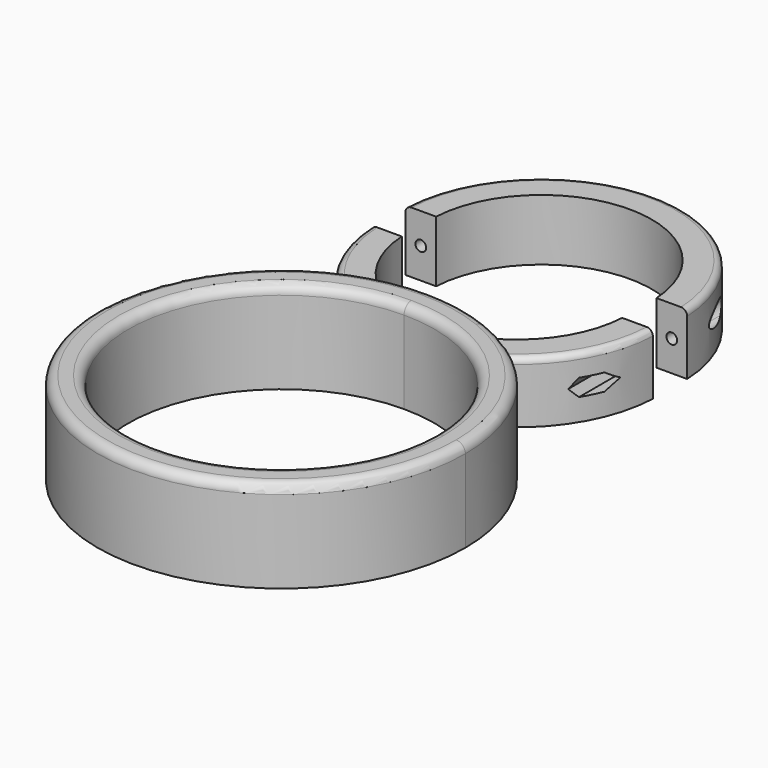
from build123d import *

# Parameters (mm, degrees)
F1_DEPTH       = 20
F2_DEPTH       = 30
F3_R           = 1.75
F4_DEPTH       = 23.9
F5_DEPTH       = 25
F6_DEPTH       = 4
F7_R           = 1.75
F8_DEPTH       = 25
F9_DEPTH       = 25
F10_DEPTH      = 7
F11_R          = 3
F12_T4_ANGLE   = 71.0644406489
F12_S5_R       = 60
F12_T6_DEPTH   = 31
F12_T10_ANGLE  = 71.0644406489
F12_S11_R      = 60
F12_T12_DEPTH  = 31
F12_2_T2_ANGLE = 187.4907274343


# Not quite as in the source:
# - a fillet or chamfer that OpenCascade refuses, or shapes differently, is made with other operations: its cross-section is extruded or revolved along the edge and cut away or added


with BuildPart() as f1:
    # F0 (on Top) → F1 (new body)
    with BuildSketch(Plane.XY):
        with BuildLine():
            ThreePointArc((-2.47e-08, 60), (11.3192314105, 58.9226187493), (22.2319585876, 55.7291666667))
            ThreePointArc((22.2319585876, 55.7291666667), (39.0970674362, 71.763265115), (45.9565011723, 94))
            Line((45.9565011723, 94), (35.9444015112, 94))
            ThreePointArc((35.9444015112, 94), (24.7386337447, 69.8466063303), (-2.47e-08, 60))
        make_face()
    extrude(amount=F1_DEPTH)



with BuildPart() as f1b:
    # F0 (on Top) → F1, piece 2 (new body)
    with BuildSketch(Plane.XY):
        with BuildLine():
            ThreePointArc((-45.9565011723, 94), (-39.0970674362, 71.763265115), (-22.2319585876, 55.7291666667))
            ThreePointArc((-22.2319585876, 55.7291666667), (-11.3192314348, 58.9226187446), (-2.47e-08, 60))
            ThreePointArc((-2.47e-08, 60), (-24.7386337627, 69.8466063473), (-35.9444015112, 94))
            Line((-35.9444015112, 94), (-45.9565011723, 94))
        make_face()
    extrude(amount=F1_DEPTH)


with BuildPart() as f1c:
    # F0 (on Top) → F1, piece 3 (new body)
    with BuildSketch(Plane.XY):
        with BuildLine():
            Line((35.9444015112, 108), (45.9565011723, 108))
            ThreePointArc((45.9565011723, 108), (0, 152), (-45.9565011723, 108))
            Line((-45.9565011723, 108), (-35.9444015112, 108))
            ThreePointArc((-35.9444015112, 108), (0, 142), (35.9444015112, 108))
        make_face()
    extrude(amount=F1_DEPTH)

    # F7 (on face) → F8 (cut)
    with BuildSketch(Plane.XZ.offset(-108)):
        with Locations((-40.9504513418, 10)):
            Circle(F7_R)
        with Locations((40.9504513418, 10)):
            Circle(F7_R)
    extrude(amount=-F8_DEPTH, mode=Mode.SUBTRACT)

    # F7 (on face) → F9 (cut)
    with BuildSketch(Plane.XZ.offset(-108)):
        with BuildLine():
            Line((-39.4004513418, 12.6846787517), (-37.8504513418, 10))
            ThreePointArc((-37.8504513418, 10), (-38.26577259, 11.55), (-39.4004513418, 12.6846787517))
        make_face()
        Polygon((-42.5004513418, 7.3153212483), (-39.4004513418, 7.3153212483), (-37.8504513418, 10), (-39.4004513418, 12.6846787517), (-42.5004513418, 12.6846787517), (-44.0504513418, 10), align=None)
        with Locations((-40.9504513418, 10)):
            Circle(F7_R, mode=Mode.SUBTRACT)
        with BuildLine():
            Line((-42.5004513418, 12.6846787517), (-39.4004513418, 12.6846787517))
            ThreePointArc((-39.4004513418, 12.6846787517), (-40.9504513418, 13.1), (-42.5004513418, 12.6846787517))
        make_face()
        with BuildLine():
            ThreePointArc((-42.5004513418, 12.6846787517), (-43.6351300935, 11.55), (-44.0504513418, 10))
            Line((-44.0504513418, 10), (-42.5004513418, 12.6846787517))
        make_face()
        with BuildLine():
            ThreePointArc((-44.0504513418, 10), (-43.6351300935, 8.45), (-42.5004513418, 7.3153212483))
            Line((-42.5004513418, 7.3153212483), (-44.0504513418, 10))
        make_face()
        with BuildLine():
            ThreePointArc((-42.5004513418, 7.3153212483), (-40.9504513418, 6.9), (-39.4004513418, 7.3153212483))
            Line((-39.4004513418, 7.3153212483), (-42.5004513418, 7.3153212483))
        make_face()
        with BuildLine():
            Line((-37.8504513418, 10), (-39.4004513418, 7.3153212483))
            ThreePointArc((-39.4004513418, 7.3153212483), (-38.26577259, 8.45), (-37.8504513418, 10))
        make_face()
        with BuildLine():
            Line((37.8504513418, 10), (39.4004513418, 12.6846787517))
            ThreePointArc((39.4004513418, 12.6846787517), (38.26577259, 11.55), (37.8504513418, 10))
        make_face()
        Polygon((44.0504513418, 10), (42.5004513418, 12.6846787517), (39.4004513418, 12.6846787517), (37.8504513418, 10), (39.4004513418, 7.3153212483), (42.5004513418, 7.3153212483), align=None)
        with Locations((40.9504513418, 10)):
            Circle(F7_R, mode=Mode.SUBTRACT)
        with BuildLine():
            Line((39.4004513418, 12.6846787517), (42.5004513418, 12.6846787517))
            ThreePointArc((42.5004513418, 12.6846787517), (40.9504513418, 13.1), (39.4004513418, 12.6846787517))
        make_face()
        with BuildLine():
            ThreePointArc((44.0504513418, 10), (43.6351300935, 11.55), (42.5004513418, 12.6846787517))
            Line((42.5004513418, 12.6846787517), (44.0504513418, 10))
        make_face()
        with BuildLine():
            ThreePointArc((42.5004513418, 7.3153212483), (43.6351300935, 8.45), (44.0504513418, 10))
            Line((44.0504513418, 10), (42.5004513418, 7.3153212483))
        make_face()
        with BuildLine():
            Line((39.4004513418, 7.3153212483), (37.8504513418, 10))
            ThreePointArc((37.8504513418, 10), (38.26577259, 8.45), (39.4004513418, 7.3153212483))
        make_face()
        with BuildLine():
            ThreePointArc((39.4004513418, 7.3153212483), (40.9504513418, 6.9), (42.5004513418, 7.3153212483))
            Line((42.5004513418, 7.3153212483), (39.4004513418, 7.3153212483))
        make_face()
    extrude(amount=-F9_DEPTH, mode=Mode.SUBTRACT)

    # F7 (on face) → F10 (join)
    with BuildSketch(Plane.XZ.offset(-108)):
        Polygon((44.0504513418, 10), (42.5004513418, 12.6846787517), (39.4004513418, 12.6846787517), (37.8504513418, 10), (39.4004513418, 7.3153212483), (42.5004513418, 7.3153212483), align=None)
        with Locations((40.9504513418, 10)):
            Circle(F7_R, mode=Mode.SUBTRACT)
        with BuildLine():
            Line((37.8504513418, 10), (39.4004513418, 12.6846787517))
            ThreePointArc((39.4004513418, 12.6846787517), (38.26577259, 11.55), (37.8504513418, 10))
        make_face()
        with BuildLine():
            Line((39.4004513418, 7.3153212483), (37.8504513418, 10))
            ThreePointArc((37.8504513418, 10), (38.26577259, 8.45), (39.4004513418, 7.3153212483))
        make_face()
        with BuildLine():
            ThreePointArc((39.4004513418, 7.3153212483), (40.9504513418, 6.9), (42.5004513418, 7.3153212483))
            Line((42.5004513418, 7.3153212483), (39.4004513418, 7.3153212483))
        make_face()
        with BuildLine():
            ThreePointArc((42.5004513418, 7.3153212483), (43.6351300935, 8.45), (44.0504513418, 10))
            Line((44.0504513418, 10), (42.5004513418, 7.3153212483))
        make_face()
        with BuildLine():
            ThreePointArc((44.0504513418, 10), (43.6351300935, 11.55), (42.5004513418, 12.6846787517))
            Line((42.5004513418, 12.6846787517), (44.0504513418, 10))
        make_face()
        with BuildLine():
            Line((39.4004513418, 12.6846787517), (42.5004513418, 12.6846787517))
            ThreePointArc((42.5004513418, 12.6846787517), (40.9504513418, 13.1), (39.4004513418, 12.6846787517))
        make_face()
        with BuildLine():
            Line((-39.4004513418, 12.6846787517), (-37.8504513418, 10))
            ThreePointArc((-37.8504513418, 10), (-38.26577259, 11.55), (-39.4004513418, 12.6846787517))
        make_face()
        Polygon((-42.5004513418, 7.3153212483), (-39.4004513418, 7.3153212483), (-37.8504513418, 10), (-39.4004513418, 12.6846787517), (-42.5004513418, 12.6846787517), (-44.0504513418, 10), align=None)
        with Locations((-40.9504513418, 10)):
            Circle(F7_R, mode=Mode.SUBTRACT)
        with BuildLine():
            Line((-37.8504513418, 10), (-39.4004513418, 7.3153212483))
            ThreePointArc((-39.4004513418, 7.3153212483), (-38.26577259, 8.45), (-37.8504513418, 10))
        make_face()
        with BuildLine():
            ThreePointArc((-42.5004513418, 7.3153212483), (-40.9504513418, 6.9), (-39.4004513418, 7.3153212483))
            Line((-39.4004513418, 7.3153212483), (-42.5004513418, 7.3153212483))
        make_face()
        with BuildLine():
            ThreePointArc((-44.0504513418, 10), (-43.6351300935, 8.45), (-42.5004513418, 7.3153212483))
            Line((-42.5004513418, 7.3153212483), (-44.0504513418, 10))
        make_face()
        with BuildLine():
            ThreePointArc((-42.5004513418, 12.6846787517), (-43.6351300935, 11.55), (-44.0504513418, 10))
            Line((-44.0504513418, 10), (-42.5004513418, 12.6846787517))
        make_face()
        with BuildLine():
            Line((-42.5004513418, 12.6846787517), (-39.4004513418, 12.6846787517))
            ThreePointArc((-39.4004513418, 12.6846787517), (-40.9504513418, 13.1), (-42.5004513418, 12.6846787517))
        make_face()
    extrude(amount=-F10_DEPTH)

    # F12#2: fillet of radius 2 on 1 edges, made by hand

    # F12_2_s1 → F12_2_t2 (revolve, cut)
    with BuildSketch(Plane(origin=(6.909384127, 105.5476965336, 0), x_dir=(0, 0, 1), z_dir=(-0.0653223839, -0.9978642123, 0))):
        with BuildLine():
            ThreePointArc((18, -39.07582731), (19.4142135624, -38.4900408724), (20, -37.07582731))
            Line((20, -37.07582731), (20, -39.07582731))
            Line((20, -39.07582731), (18, -39.07582731))
        make_face()
    revolve(axis=Axis((0, 106, 20), (0, 0, 1)), revolution_arc=F12_2_T2_ANGLE, mode=Mode.SUBTRACT)


with BuildPart() as f1_1:
    add(f1.part)

    add(f1b.part)  # F2 merges F1b
    # F0 (on Top) → F2 (join)
    with BuildSketch(Plane.XY):
        with BuildLine():
            ThreePointArc((22.2319585876, 55.7291666667), (11.4791477819, 51.4553127051), (4.18e-08, 50))
            ThreePointArc((4.18e-08, 50), (-11.4791477414, 51.4553126946), (-22.2319585876, 55.7291666667))
            ThreePointArc((-22.2319585876, 55.7291666667), (-33.6606779845, -49.668488578), (60, 0))
            ThreePointArc((60, 0), (49.668488578, 33.6606779845), (22.2319585876, 55.7291666667))
        make_face()
        with BuildLine():
            ThreePointArc((4.18e-08, 50), (35.3553390741, 35.3553390445), (50, 0))
            ThreePointArc((50, 0), (-35.3553390741, -35.3553390445), (4.18e-08, 50))
        make_face(mode=Mode.SUBTRACT)
        with BuildLine():
            ThreePointArc((-22.2319585876, 55.7291666667), (-11.4791477414, 51.4553126946), (4.18e-08, 50))
            ThreePointArc((4.18e-08, 50), (11.4791477819, 51.4553127051), (22.2319585876, 55.7291666667))
            ThreePointArc((22.2319585876, 55.7291666667), (11.3192314105, 58.9226187493), (-2.47e-08, 60))
            ThreePointArc((-2.47e-08, 60), (-11.3192314348, 58.9226187446), (-22.2319585876, 55.7291666667))
        make_face()
    extrude(amount=F2_DEPTH)

    # F3 (on face) → F4 (cut)
    with BuildSketch(Plane(origin=(0, 94, 0), x_dir=(-1, 0, 0), z_dir=(0, 1, 0))):
        with Locations((-40.9504513418, 10)):
            Circle(F3_R)
        with Locations((40.9504513418, 10)):
            Circle(F3_R)
    extrude(amount=-F4_DEPTH, mode=Mode.SUBTRACT)

    # F3 (on face) → F5 (cut)
    with BuildSketch(Plane(origin=(0, 94, 0), x_dir=(-1, 0, 0), z_dir=(0, 1, 0))):
        Polygon((-42.5504513418, 7.2287187079), (-39.3504513418, 7.2287187079), (-37.7504513418, 10), (-39.3504513418, 12.7712812921), (-42.5504513418, 12.7712812921), (-44.1504513418, 10), align=None)
        with Locations((-40.9504513418, 10)):
            Circle(F3_R, mode=Mode.SUBTRACT)
        Polygon((42.5504513418, 12.7712812921), (39.3504513418, 12.7712812921), (37.7504513418, 10), (39.3504513418, 7.2287187079), (42.5504513418, 7.2287187079), (44.1504513418, 10), align=None)
        with Locations((40.9504513418, 10)):
            Circle(F3_R, mode=Mode.SUBTRACT)
    extrude(amount=-F5_DEPTH, mode=Mode.SUBTRACT)

    # F3 (on face) → F6 (join)
    with BuildSketch(Plane(origin=(0, 94, 0), x_dir=(-1, 0, 0), z_dir=(0, 1, 0))):
        Polygon((-42.5504513418, 7.2287187079), (-39.3504513418, 7.2287187079), (-37.7504513418, 10), (-39.3504513418, 12.7712812921), (-42.5504513418, 12.7712812921), (-44.1504513418, 10), align=None)
        with Locations((-40.9504513418, 10)):
            Circle(F3_R, mode=Mode.SUBTRACT)
        Polygon((42.5504513418, 12.7712812921), (39.3504513418, 12.7712812921), (37.7504513418, 10), (39.3504513418, 7.2287187079), (42.5504513418, 7.2287187079), (44.1504513418, 10), align=None)
        with Locations((40.9504513418, 10)):
            Circle(F3_R, mode=Mode.SUBTRACT)
    extrude(amount=-F6_DEPTH)

    # F11
    f11_edges = [f1_1.edges().sort_by_distance(p)[0] for p in [
        (-22.231959, -55.729167, 30),
        (0, -50, 30),
    ]]
    fillet(f11_edges, radius=F11_R)

    # F12: fillet of radius 2 on 2 edges, made by hand


with BuildPart() as f12_tool2:
    # F12_s3 → F12_t4 (revolve)
    with BuildSketch(Plane(origin=(34.1449001636, 14.2638799975, 0), x_dir=(0, 0, 1), z_dir=(-0.9227230986, -0.3854634656, 0))):
        with BuildLine():
            ThreePointArc((18, 42.5814174657), (19.4142135624, 43.1672039033), (20, 44.5814174657))
            Line((20, 44.5814174657), (20, 42.5814174657))
            Line((20, 42.5814174657), (18, 42.5814174657))
        make_face()
    revolve(axis=Axis((0, 96, 20), (0, 0, 1)), revolution_arc=F12_T4_ANGLE)

    # F12_s5 → F12_t6 (cut, symmetric)
    with BuildSketch(Plane.XY.offset(19)):
        Circle(F12_S5_R)
    extrude(amount=F12_T6_DEPTH, both=True, mode=Mode.SUBTRACT)


with BuildPart() as f1_2:
    add(f1_1.part)

    # F12_t1: cut F12_tool2
    add(f12_tool2.part, mode=Mode.SUBTRACT)


with BuildPart() as f12_tool8:
    # F12_s9 → F12_t10 (revolve)
    with BuildSketch(Plane(origin=(6.243588842, 95.5922010247, 0), x_dir=(0, 0, 1), z_dir=(0.0651759618, 0.9978737866, 0))):
        with BuildLine():
            ThreePointArc((18, -52.2568923302), (19.4142135624, -51.6711058926), (20, -50.2568923302))
            Line((20, -50.2568923302), (20, -52.2568923302))
            Line((20, -52.2568923302), (18, -52.2568923302))
        make_face()
    revolve(axis=Axis((0, 96, 20), (0, 0, 1)), revolution_arc=F12_T10_ANGLE)

    # F12_s11 → F12_t12 (cut, symmetric)
    with BuildSketch(Plane.XY.offset(19)):
        Circle(F12_S11_R)
    extrude(amount=F12_T12_DEPTH, both=True, mode=Mode.SUBTRACT)


with BuildPart() as f1_3:
    add(f1_2.part)

    # F12_t7: cut F12_tool8
    add(f12_tool8.part, mode=Mode.SUBTRACT)


solid = Compound([f1c.part, f1_3.part])
